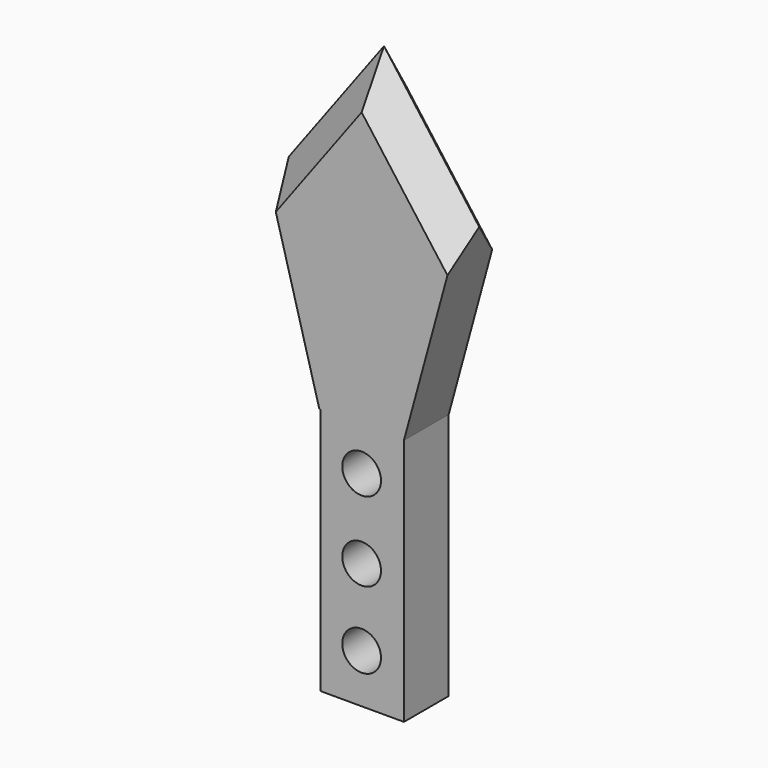
from build123d import *

# Parameters (mm, degrees)
F0_W     = 18.9141826704
F0_H     = 56.2922134995
F1_DEPTH = 12.7
F3_D     = 8.8
F5_DEPTH = 12.7
F6_SIZE  = 6.34999


# Not quite as in the source:
# - a fillet or chamfer is up to 0.001 mm smaller than in the source, because OpenCascade refuses the exact size


with BuildPart() as f1:
    # F0 (on Front) → F1 (new body)
    with BuildSketch(Plane.XZ):
        with Locations((0.1501129009, -28.1461067498)):
            Rectangle(F0_W, F0_H)
    extrude(amount=F1_DEPTH)

    # F3 (through all)
    with Locations(Plane(origin=(0, 0, 0), x_dir=(1, 0, 0), z_dir=(0, 1, 0))):
        with Locations((0, 9.7573176026), (0, 27.770826593), (0, 45.1838858426)):
            Hole(F3_D / 2)

    # F4 (on Front) → F5 (join)
    with BuildSketch(Plane.XZ):
        Polygon((0, 0), (9.6072051674, 0), (21.6162092984, 43.9829826355), (0, 73.1048211455), (-21.6162092984, 43.9829826355), (-9.6072051674, 0), align=None)
    extrude(amount=F5_DEPTH)

    # F6 (size 6.35 in the source; OpenCascade refuses exactly that, so slightly less here)
    f6_edges = [f1.edges().sort_by_distance(p)[0] for p in [
        (10.808105, 0, 58.543902),
        (-10.808105, 0, 58.543902),
        (10.808105, -12.7, 58.543902),
        (-10.808105, -12.7, 58.543902),
    ]]
    chamfer(f6_edges, length=F6_SIZE)


solid = f1.part
